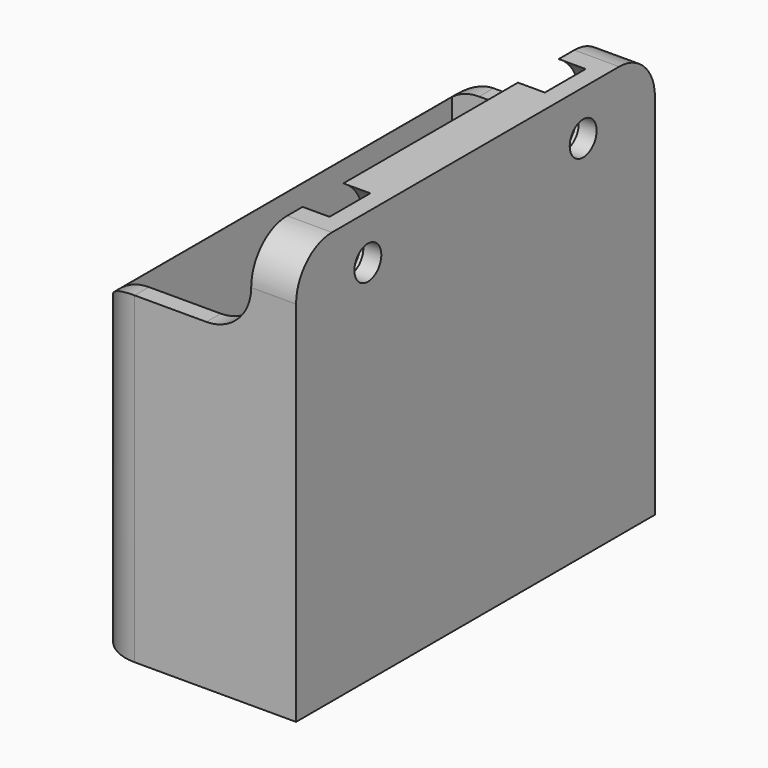
from build123d import *

# Parameters (mm, degrees)
F0_W        = 20
F0_H        = 50
F0_W_2      = 16
F0_H_2      = 46
F1_DEPTH    = 2
F2_DEPTH    = 36
F4_DEPTH    = 10
F5_R        = 1.875
F6_DEPTH    = 25
F7_T1_DEPTH = 2
F7_T3_DEPTH = 2
F7_T5_DEPTH = 61
F7_T7_DEPTH = 27
F7_T9_DEPTH = 75
F8_DEPTH    = 3
F9_DEPTH    = 3


# Not quite as in the source:
# - a fillet or chamfer that OpenCascade refuses, or shapes differently, is made with other operations: its cross-section is extruded or revolved along the edge and cut away or added


with BuildPart() as f1:
    # F0 (on Top) → F1 (new body)
    with BuildSketch(Plane.XY):
        Rectangle(F0_W, F0_H)
        Rectangle(F0_W_2, F0_H_2, mode=Mode.SUBTRACT)
        Rectangle(F0_W_2, F0_H_2)
    extrude(amount=F1_DEPTH)

    # F0 (on Top) → F2 (join)
    with BuildSketch(Plane.XY):
        Rectangle(F0_W, F0_H)
        Rectangle(F0_W_2, F0_H_2, mode=Mode.SUBTRACT)
    extrude(amount=F2_DEPTH)

    # F3 (on face) → F4 (join)
    with BuildSketch(Plane.XY.offset(36)):
        Polygon((10, -25), (10, 25), (8, 25), (8, 23), (8, -23), (8, -25), align=None)
    extrude(amount=F4_DEPTH)

    # F5 (on face) → F6 (cut)
    with BuildSketch(Plane(origin=(8, 0, 0), x_dir=(0, -1, 0), z_dir=(-1, 0, 0))):
        with Locations((15, 41)):
            Circle(F5_R)
        with Locations((-15, 41)):
            Circle(F5_R)
    extrude(amount=-F6_DEPTH, mode=Mode.SUBTRACT)

    # F7: fillet of radius 5 on 7 edges, made by hand

    # F7_s2 → F7_t1 (join)
    with BuildSketch(Plane.XZ.offset(23)):
        with BuildLine():
            ThreePointArc((8, 41), (6.5355339059, 37.4644660941), (3, 36))
            Line((3, 36), (8, 36))
            Line((8, 36), (8, 41))
        make_face()
    extrude(amount=F7_T1_DEPTH)

    # F7_s4 → F7_t3 (join)
    with BuildSketch(Plane.XZ.offset(-25)):
        with BuildLine():
            ThreePointArc((8, 41), (6.5355339059, 37.4644660941), (3, 36))
            Line((3, 36), (8, 36))
            Line((8, 36), (8, 41))
        make_face()
    extrude(amount=F7_T3_DEPTH)

    # F7_s6 → F7_t5 (cut)
    with BuildSketch(Plane.XY.offset(-12.5)):
        with BuildLine():
            ThreePointArc((-5, -25), (-8.5355339059, -23.5355339059), (-10, -20))
            Line((-10, -20), (-10, -25))
            Line((-10, -25), (-5, -25))
        make_face()
        with BuildLine():
            ThreePointArc((-5, 25), (-8.5355339059, 23.5355339059), (-10, 20))
            Line((-10, 20), (-10, 25))
            Line((-10, 25), (-5, 25))
        make_face()
    extrude(amount=F7_T5_DEPTH, mode=Mode.SUBTRACT)

    # F7_s8 → F7_t7 (cut)
    with BuildSketch(Plane.YZ.offset(-4.5)):
        with BuildLine():
            ThreePointArc((-25, 41), (-23.5355339059, 44.5355339059), (-20, 46))
            Line((-20, 46), (-25, 46))
            Line((-25, 46), (-25, 41))
        make_face()
        with BuildLine():
            ThreePointArc((25, 41), (23.5355339059, 44.5355339059), (20, 46))
            Line((20, 46), (25, 46))
            Line((25, 46), (25, 41))
        make_face()
    extrude(amount=F7_T7_DEPTH, mode=Mode.SUBTRACT)

    # F7_s10 → F7_t9 (cut)
    with BuildSketch(Plane.XZ.offset(-37.5)):
        with BuildLine():
            ThreePointArc((-10, 31), (-8.5355339059, 34.5355339059), (-5, 36))
            Line((-5, 36), (-10, 36))
            Line((-10, 36), (-10, 31))
        make_face()
    extrude(amount=F7_T9_DEPTH, mode=Mode.SUBTRACT)

    # F8 (add): a face of the model
    f8_faces = [f1.faces().sort_by_distance(p)[0] for p in [
        (10, 0, 22.721056124),
    ]]
    extrude(f8_faces, amount=F8_DEPTH)

    # F5 (on face) → F9 (cut)
    with BuildSketch(Plane(origin=(8, 0, 0), x_dir=(0, -1, 0), z_dir=(-1, 0, 0))):
        with BuildLine():
            ThreePointArc((-9.25, 41), (-10.0306257188, 43.8927183155), (-12.1605458271, 46))
            Line((-12.1605458271, 46), (-17.8394541729, 46))
            ThreePointArc((-17.8394541729, 46), (-17.8927183155, 36.0306257188), (-9.25, 41))
        make_face()
        with Locations((-15, 41)):
            Circle(F5_R, mode=Mode.SUBTRACT)
        with BuildLine():
            ThreePointArc((12.1605458271, 46), (12.1072816845, 36.0306257188), (20.75, 41))
            ThreePointArc((20.75, 41), (19.9693742812, 43.8927183155), (17.8394541729, 46))
            Line((17.8394541729, 46), (12.1605458271, 46))
        make_face()
        with Locations((15, 41)):
            Circle(F5_R, mode=Mode.SUBTRACT)
    extrude(amount=-F9_DEPTH, mode=Mode.SUBTRACT)


solid = f1.part
